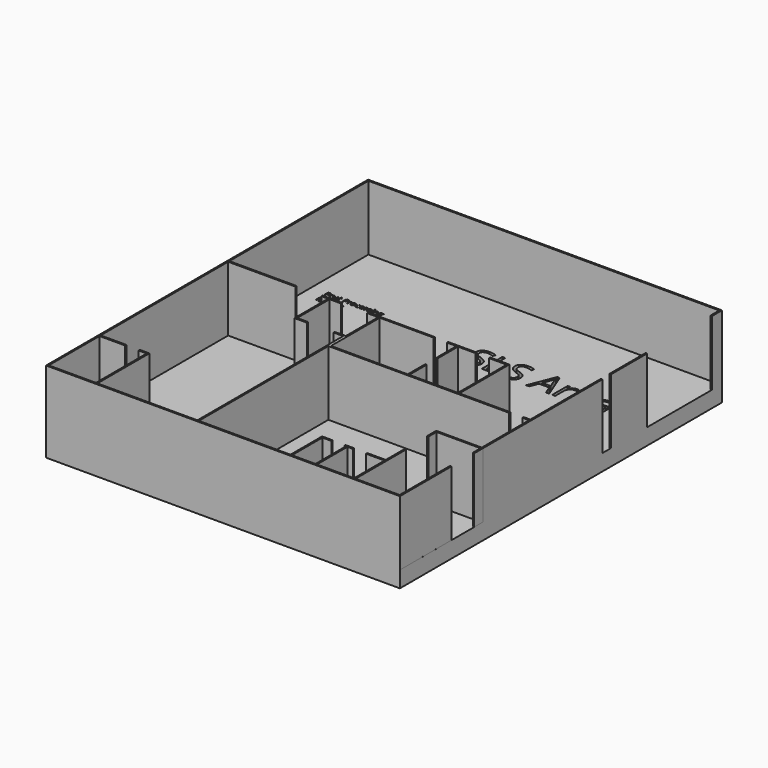
from build123d import *

# Parameters (mm, degrees)
F0_W            = 21800
F0_H            = 24800
F1_DEPTH        = 1000
F3_W            = 4730
F3_H            = 3755.5469703674
F3_W_2          = 3000
F4_DEPTH        = 4000
F5_W            = 3000
F5_H            = 2500
F6_DEPTH        = 4000
F8_DEPTH        = 4000
F9_W            = 820
F9_H            = 90
F9_W_2          = 90
F9_H_2          = 820
F9_W_3          = 1640
F9_W_4          = 1620
F10_DEPTH       = 4000
F11_TEXT_SIZE   = 1027.7540967842
F11_TEXT_SIZE_2 = 2229.5511510536
F11_TEXT_SIZE_3 = 488.0318210498
F12_DEPTH       = 500
F13_W           = 1450
F13_H           = 2347.1213800322
F13_W_2         = 2290
F13_W_3         = 2715
F13_H_2         = 6235
F14_DEPTH       = 4000
F15_W           = 700
F15_H           = 2527.1213800322
F16_DEPTH       = 1250
F17_W           = 5645
F17_H           = 90
F18_DEPTH       = 4000
F19_W           = 90
F19_H           = 1750
F19_H_2         = 5000
F19_H_3         = 650
F19_W_2         = 800
F19_H_4         = 90
F20_DEPTH       = 4000
F22_W           = 1600
F22_H           = 90
F23_DEPTH       = 4000
F25_DEPTH       = 4000


# Not quite as in the source:
# - Text() gives the source's letters only with a copy of the font that has no kerning and outlines rounded to 1/6400 em; it was checked with that copy


with BuildPart() as f1:
    # F0 (on Top) → F1 (new body)
    with BuildSketch(Plane.XY):
        Rectangle(F0_W, F0_H)
    extrude(amount=F1_DEPTH)

    # F3 (on face) → F4 (join)
    with BuildSketch(Plane.XY.offset(1000)):
        Polygon((6439.6429443359, 1600), (-1560.3570556641, 1600), (-1560.3570556641, -400), (-1560.3570556641, -2335.5469703674), (6439.6429443359, -2335.5469703674), (10899.2567062378, -2335.5469703674), (10899.2567062378, -2245.5469703674), (6439.6429443359, -2245.5469703674), align=None)
        with Locations((894.6429443359, -367.7734851837)):
            Rectangle(F3_W, F3_H, mode=Mode.SUBTRACT)
        with Locations((4849.6429443359, -367.7734851837)):
            Rectangle(F3_W_2, F3_H, mode=Mode.SUBTRACT)
        Polygon((-1560.3570556641, -400), (-1560.3570556641, 1600), (-4560.3570556641, 1600), (-10900, 1600), (-10900, -12400), (-4560.3570556641, -12400), (-1560.3570556641, -12400), (-1560.3570556641, -9400), (-1560.3570556641, -2335.5469703674), align=None)
    extrude(amount=F4_DEPTH)

    # F5 (on face) → F6 (cut)
    with BuildSketch(Plane.XY.offset(5000)):
        with Locations((-3060.3570556641, 260)):
            Rectangle(F5_W, F5_H)
    extrude(amount=-F6_DEPTH, mode=Mode.SUBTRACT)

    # F7 (on face) → F8 (cut)
    with BuildSketch(Plane.XY.offset(5000)):
        Polygon((-4650.3570556641, -1080), (-4650.3570556641, 1510), (-10810, 1510), (-10810, -8310), (-7810, -8310), (-7810, -12310), (-4650.3570556641, -12310), (-1650.3570556641, -12310), (-1650.3570556641, -9220), (-1650.3570556641, -1080), align=None)
    extrude(amount=-F8_DEPTH, mode=Mode.SUBTRACT)

    # F9 (on face) → F10 (cut)
    with BuildSketch(Plane.XY.offset(5000)):
        with Locations((2259.6429443359, 1555)):
            Rectangle(F9_W, F9_H)
        with Locations((3304.6429443359, -490)):
            Rectangle(F9_W_2, F9_H_2)
        with Locations((4849.6429443359, 1555)):
            Rectangle(F9_W, F9_H)
        with Locations((9989.6429443359, -2290.5469703674)):
            Rectangle(F9_W, F9_H)
        with Locations((-3060.3570556641, -1035)):
            Rectangle(F9_W_3, F9_H)
        with Locations((-3060.3570556641, 1555)):
            Rectangle(F9_W_4, F9_H)
        with Locations((-8820, -8355)):
            Rectangle(F9_W, F9_H)
    extrude(amount=-F10_DEPTH, mode=Mode.SUBTRACT)

    # F11 (on face) → F12 (cut)
    with BuildSketch(Plane.XY.offset(1000)):
        with Locations((-560.3570556641, -7092.7375420983)):
            Text('Breakout Room', F11_TEXT_SIZE, font='Open Sans', text_align=(TextAlign.LEFT, TextAlign.BOTTOM))
        with Locations((-560.3570556641, 6423.0970558727)):
            Text('SLS Area', F11_TEXT_SIZE_2, font='Open Sans', text_align=(TextAlign.LEFT, TextAlign.BOTTOM))
        with Locations((-9900, 7676.9909734754)):
            Text('Post Processing', F11_TEXT_SIZE_3, font='Open Sans', text_align=(TextAlign.LEFT, TextAlign.BOTTOM))
        with Locations((-9900, 7013.2676968477)):
            Text('for SLS', F11_TEXT_SIZE_3, font='Open Sans', text_align=(TextAlign.LEFT, TextAlign.BOTTOM))
    extrude(amount=-F12_DEPTH, mode=Mode.SUBTRACT)

    # F13 (on face) → F14 (join)
    with BuildSketch(Plane.XY.offset(1000)):
        Polygon((10899.6429443359, -12400), (10899.6429443359, -5985), (8004.6429443359, -5985), (8004.6429443359, -9872.8786199678), (4084.6429443359, -9872.8786199678), (4084.6429443359, -12400), (8004.6429443359, -12400), (8701.4996466017, -12400), align=None)
        with Locations((4899.6429443359, -11136.4393099839)):
            Rectangle(F13_W, F13_H, mode=Mode.SUBTRACT)
        with Locations((6859.6429443359, -11136.4393099839)):
            Rectangle(F13_W_2, F13_H, mode=Mode.SUBTRACT)
        with Locations((9452.1429443359, -9192.5)):
            Rectangle(F13_W_3, F13_H_2, mode=Mode.SUBTRACT)
    extrude(amount=F14_DEPTH)

    # F15 (on face) → F16 (join)
    with BuildSketch(Plane.XY.offset(1000)):
        with Locations((3734.6429443359, -11136.4393099839)):
            Rectangle(F15_W, F15_H)
    extrude(amount=F16_DEPTH)

    # F17 (on face) → F18 (join)
    with BuildSketch(Plane.XY.offset(1000)):
        Polygon((-10900, 12400), (-10900, 1600), (-10810, 1600), (-10810, 12310), (10810, 12310), (10810, -5985), (10900, -5985), (10900, 12310), (10900, 12400), (-10810, 12400), align=None)
        with Locations((1262.1429443359, -12355)):
            Rectangle(F17_W, F17_H)
    extrude(amount=F18_DEPTH)

    # F19 (on face) → F20 (cut)
    with BuildSketch(Plane.XY.offset(5000)):
        with Locations((10854.6429443359, -7550)):
            Rectangle(F19_W, F19_H)
        with Locations((10855, 9135)):
            Rectangle(F19_W, F19_H_2)
        with Locations((10855, 3515)):
            Rectangle(F19_W, F19_H_3)
        with Locations((8049.6429443359, -7550)):
            Rectangle(F19_W, F19_H)
        with Locations((6459.6429443359, -9917.8786199678)):
            Rectangle(F19_W_2, F19_H_4)
        with Locations((5124.6429443359, -9917.8786199678)):
            Rectangle(F19_W_2, F19_H_4)
    extrude(amount=-F20_DEPTH, mode=Mode.SUBTRACT)

    # F22 (on face) → F23 (cut)
    with BuildSketch(Plane.XY.offset(5000)):
        with Locations((-5869.4512367249, 1555)):
            Rectangle(F22_W, F22_H)
    extrude(amount=-F23_DEPTH, mode=Mode.SUBTRACT)

    # F24 (on face) → F25 (cut)
    with BuildSketch(Plane.XY.offset(5000)):
        Polygon((-10810.0004196167, -8400), (-10810.0004196167, -12310), (-7900.0004196167, -12310), (-7900.0004196167, -8400), (-8410, -8400), (-9230, -8400), align=None)
    extrude(amount=-F25_DEPTH, mode=Mode.SUBTRACT)


solid = f1.part
